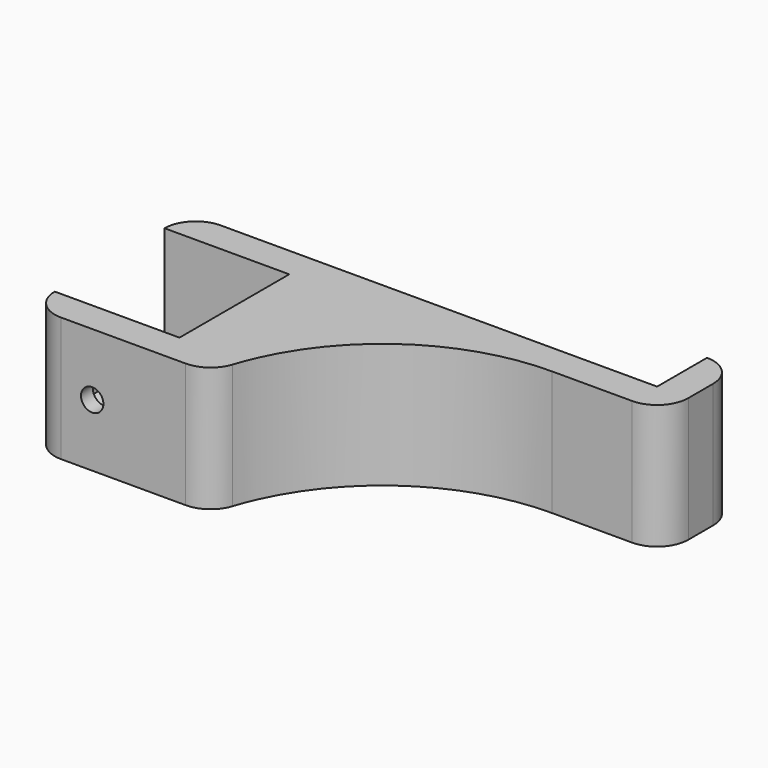
from build123d import *

# Parameters (mm, degrees)
F3_DEPTH = 20
F4_R     = 4.99999
F6_DEPTH = 2.6
F7_D     = 3.6
F7_DEPTH = 10
F7_TIP   = 1.0815491142
F8_R     = 34


# Not quite as in the source:
# - a fillet or chamfer is up to 0.001 mm smaller than in the source, because OpenCascade refuses the exact size


with BuildPart() as f3:
    # F2 (on Top) → F3 (new body)
    with BuildSketch(Plane.XY):
        Polygon((0, 5), (0, 0), (20, 0), (20, -22), (0, -22), (0, -27), (30, -27), (30, 0), (80, 0), (80, 15), (75, 15), (75, 5), align=None)
    extrude(amount=F3_DEPTH)

    # F4 (radius 5 in the source; OpenCascade refuses exactly that, so slightly less here)
    f4_edges = [f3.edges().sort_by_distance(p)[0] for p in [
        (30, -27, 10),
        (80, 0, 10),
        (80, 15, 10),
        (0, 5, 10),
        (0, -27, 10),
    ]]
    fillet(f4_edges, radius=F4_R)

    # F5 (on face) → F6 (cut)
    with BuildSketch(Plane(origin=(0, -22, 0), x_dir=(-1, 0, 0), z_dir=(0, 1, 0))):
        Polygon((-7.25, 8.4122867597), (-7.25, 11.5877132403), (-10, 13.1754264805), (-12.75, 11.5877132403), (-12.75, 8.4122867597), (-10, 6.8245735195), align=None)
    extrude(amount=-F6_DEPTH, mode=Mode.SUBTRACT)

    # F7 (one way)
    with BuildSketch(Plane(origin=(0, -22, 0), x_dir=(-1, 0, 0), z_dir=(0, 1, 0))):
        with Locations((-10, 10)):
            Circle(F7_D / 2)
    extrude(amount=-F7_DEPTH, mode=Mode.SUBTRACT)
    with Locations(Plane(origin=(0, -22, 0), x_dir=(-1, 0, 0), z_dir=(0, 1, 0))):
        with Locations((-10, 10)):
            with Locations((0, 0, -(F7_DEPTH + F7_TIP / 2))):  # 118° drill point
                Cone(0, F7_D / 2, F7_TIP, mode=Mode.SUBTRACT)

    # F8
    f8_edges = [f3.edges().sort_by_distance(p)[0] for p in [
        (30, 0, 10),
    ]]
    fillet(f8_edges, radius=F8_R)


solid = f3.part
